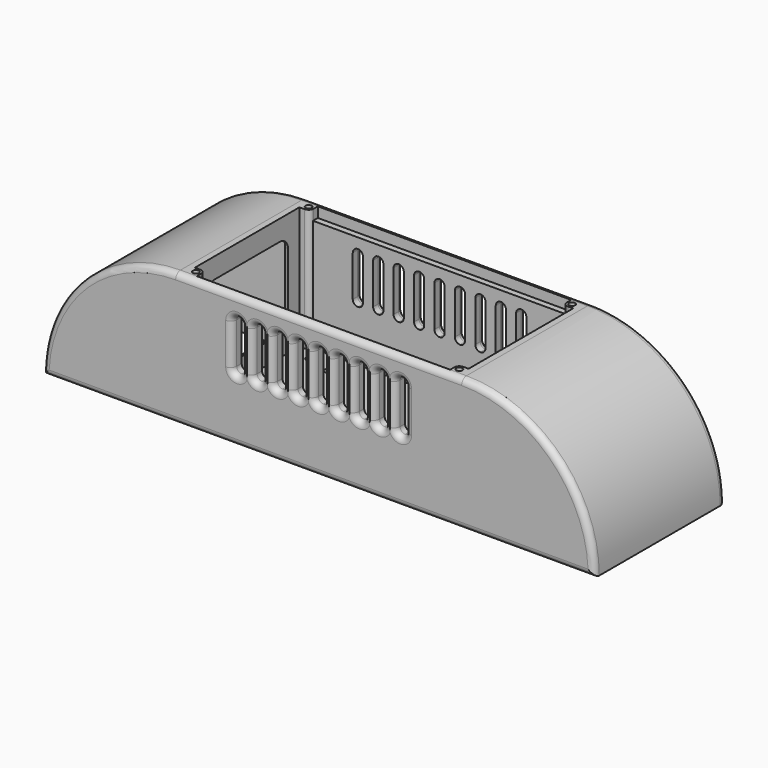
from build123d import *

# Parameters (mm, degrees)
F0_R           = 2.5
F0_R_2         = 1.5
F1_DEPTH       = 5
F0_W           = 140
F0_H           = 80
F2_DEPTH       = 65
F5_DEPTH       = 10
F8_DEPTH       = 10
F9_DEPTH       = 60
F10_DEPTH      = 85
F13_DEPTH      = 80
F14_DEPTH      = 70
F15_T1_DEPTH   = 70
F15_T3_DEPTH   = 285
F15_T5_DEPTH   = 140
F15_T7_DEPTH   = 20
F15_T9_DEPTH   = 70
F15_T11_DEPTH  = 46
F15_T13_DEPTH  = 40
F15_T15_DEPTH  = 30
F15_T17_DEPTH  = 27.5
F15_T20_ANGLE  = 96.6137071956
F15_T22_ANGLE  = 96.6137071956
F15_T24_ANGLE  = 96.6137071956
F15_T26_ANGLE  = 180
F15_T28_ANGLE  = 180
F15_T30_ANGLE  = 180
F15_T32_ANGLE  = 180
F15_T34_ANGLE  = 180
F15_T36_ANGLE  = 180
F15_T38_ANGLE  = 180
F15_T40_ANGLE  = 180
F15_T42_ANGLE  = 180
F15_T44_ANGLE  = 180
F15_T46_ANGLE  = 180
F15_T48_ANGLE  = 180
F15_T50_ANGLE  = 180
F15_T52_ANGLE  = 180
F15_T54_ANGLE  = 180
F15_T56_ANGLE  = 180
F15_T58_ANGLE  = 180
F15_T60_ANGLE  = 180
F15_T62_ANGLE  = 96.6137071956
F15_T64_ANGLE  = 180
F15_T66_ANGLE  = 180
F15_T68_ANGLE  = 180
F15_T70_ANGLE  = 180
F15_T72_ANGLE  = 180
F15_T74_ANGLE  = 180
F15_T76_ANGLE  = 180
F15_T78_ANGLE  = 180
F15_T80_ANGLE  = 180
F15_T82_ANGLE  = 180
F15_T84_ANGLE  = 180
F15_T86_ANGLE  = 180
F15_T88_ANGLE  = 180
F15_T90_ANGLE  = 180
F15_T92_ANGLE  = 180
F15_T94_ANGLE  = 180
F15_T96_ANGLE  = 180
F15_T98_ANGLE  = 180
F15_T100_ANGLE = 90
F15_T102_ANGLE = 90
F15_T104_ANGLE = 90
F15_T106_ANGLE = 90
F15_T108_ANGLE = 90
F15_T110_ANGLE = 90
F15_T112_ANGLE = 90
F15_T114_ANGLE = 90


# Not quite as in the source:
# - a fillet or chamfer that OpenCascade refuses, or shapes differently, is made with other operations: its cross-section is extruded or revolved along the edge and cut away or added


with BuildPart() as f1:
    # F0 (on Top) → F1 (new body)
    with BuildSketch(Plane.XY):
        with BuildLine():
            Line((5.5, 72), (3, 72))
            Line((3, 72), (3, 8))
            Line((3, 8), (5.5, 8))
            ThreePointArc((5.5, 8), (7.0811388301, 7.4364916731), (7.9494897428, 6))
            Line((7.9494897428, 6), (132.0505102572, 6))
            ThreePointArc((132.0505102572, 6), (132.9188611699, 7.4364916731), (134.5, 8))
            Line((134.5, 8), (137, 8))
            Line((137, 8), (137, 72))
            Line((137, 72), (134.5, 72))
            ThreePointArc((134.5, 72), (132.9188611699, 72.5635083269), (132.0505102572, 74))
            Line((132.0505102572, 74), (7.9494897428, 74))
            ThreePointArc((7.9494897428, 74), (7.0811388301, 72.5635083269), (5.5, 72))
        make_face()
        with Locations((13, 13)):
            Circle(F0_R, mode=Mode.SUBTRACT)
        with Locations((31, 15)):
            Circle(F0_R_2, mode=Mode.SUBTRACT)
        with Locations((106, 15)):
            Circle(F0_R_2, mode=Mode.SUBTRACT)
        with Locations((127, 13)):
            Circle(F0_R, mode=Mode.SUBTRACT)
        with Locations((13, 67)):
            Circle(F0_R, mode=Mode.SUBTRACT)
        with Locations((24, 63)):
            Circle(F0_R_2, mode=Mode.SUBTRACT)
        with Locations((106, 63)):
            Circle(F0_R_2, mode=Mode.SUBTRACT)
        with Locations((127, 67)):
            Circle(F0_R, mode=Mode.SUBTRACT)
    extrude(amount=F1_DEPTH)

    # F0 (on Top) → F2 (join)
    with BuildSketch(Plane.XY):
        with Locations((70, 40)):
            Rectangle(F0_W, F0_H)
        with Locations((5.5, 5.5)):
            Circle(F0_R_2, mode=Mode.SUBTRACT)
        with Locations((134.5, 5.5)):
            Circle(F0_R_2, mode=Mode.SUBTRACT)
        with Locations((5.5, 74.5)):
            Circle(F0_R_2, mode=Mode.SUBTRACT)
        with BuildLine():
            Line((3, 8), (3, 72))
            Line((3, 72), (5.5, 72))
            ThreePointArc((5.5, 72), (7.0811388301, 72.5635083269), (7.9494897428, 74))
            ThreePointArc((7.9494897428, 74), (7.9873403825, 74.248727595), (8, 74.5))
            Line((8, 74.5), (8, 77))
            Line((8, 77), (132, 77))
            Line((132, 77), (132, 74.5))
            ThreePointArc((132, 74.5), (132.0126596175, 74.248727595), (132.0505102572, 74))
            ThreePointArc((132.0505102572, 74), (132.9188611699, 72.5635083269), (134.5, 72))
            Line((134.5, 72), (137, 72))
            Line((137, 72), (137, 8))
            Line((137, 8), (134.5, 8))
            ThreePointArc((134.5, 8), (132.9188611699, 7.4364916731), (132.0505102572, 6))
            ThreePointArc((132.0505102572, 6), (132.0126596175, 5.751272405), (132, 5.5))
            Line((132, 5.5), (132, 3))
            Line((132, 3), (8, 3))
            Line((8, 3), (8, 5.5))
            ThreePointArc((8, 5.5), (7.9873403825, 5.751272405), (7.9494897428, 6))
            ThreePointArc((7.9494897428, 6), (7.0811388301, 7.4364916731), (5.5, 8))
            Line((5.5, 8), (3, 8))
        make_face(mode=Mode.SUBTRACT)
        with Locations((134.5, 74.5)):
            Circle(F0_R_2, mode=Mode.SUBTRACT)
    extrude(amount=F2_DEPTH)

    # F4 (on Right) → F5 (cut)
    with BuildSketch(Plane.YZ):
        with BuildLine():
            Line((60, 55), (20, 55))
            ThreePointArc((20, 55), (16.4644660941, 53.5355339059), (15, 50))
            Line((15, 50), (15, 20))
            ThreePointArc((15, 20), (16.4644660941, 16.4644660941), (20, 15))
            Line((20, 15), (60, 15))
            ThreePointArc((60, 15), (63.5355339059, 16.4644660941), (65, 20))
            Line((65, 20), (65, 50))
            ThreePointArc((65, 50), (63.5355339059, 53.5355339059), (60, 55))
        make_face()
    extrude(amount=F5_DEPTH, mode=Mode.SUBTRACT)

    # F7 (on offset) → F8 (cut)
    with BuildSketch(Plane.YZ.offset(140)):
        with BuildLine():
            ThreePointArc((66, 10.5), (67.4142135624, 11.0857864376), (68, 12.5))
            Line((68, 12.5), (68, 40))
            ThreePointArc((68, 40), (67.4142135624, 41.4142135624), (66, 42))
            Line((66, 42), (20, 42))
            ThreePointArc((20, 42), (18.5857864376, 41.4142135624), (18, 40))
            Line((18, 40), (18, 12.5))
            ThreePointArc((18, 12.5), (18.5857864376, 11.0857864376), (20, 10.5))
            Line((20, 10.5), (66, 10.5))
        make_face()
    extrude(amount=-F8_DEPTH, mode=Mode.SUBTRACT)

    # F0 (on Top) → F9 (join)
    with BuildSketch(Plane.XY):
        with BuildLine():
            Line((132.0505102572, 6), (7.9494897428, 6))
            ThreePointArc((7.9494897428, 6), (7.9873403825, 5.751272405), (8, 5.5))
            Line((8, 5.5), (8, 3))
            Line((8, 3), (132, 3))
            Line((132, 3), (132, 5.5))
            ThreePointArc((132, 5.5), (132.0126596175, 5.751272405), (132.0505102572, 6))
        make_face()
        with BuildLine():
            ThreePointArc((8, 74.5), (7.9873403825, 74.248727595), (7.9494897428, 74))
            Line((7.9494897428, 74), (132.0505102572, 74))
            ThreePointArc((132.0505102572, 74), (132.0126596175, 74.248727595), (132, 74.5))
            Line((132, 74.5), (132, 77))
            Line((132, 77), (8, 77))
            Line((8, 77), (8, 74.5))
        make_face()
    extrude(amount=F9_DEPTH)

    # F3 (on Front) → F10 (cut)
    with BuildSketch(Plane.XZ):
        with BuildLine():
            ThreePointArc((30, 30), (31.767766953, 30.732233047), (32.5, 32.5))
            Line((32.5, 32.5), (32.5, 52.5))
            ThreePointArc((32.5, 52.5), (31.767766953, 54.267766953), (30, 55))
            ThreePointArc((30, 55), (28.232233047, 54.267766953), (27.5, 52.5))
            Line((27.5, 52.5), (27.5, 32.5))
            ThreePointArc((27.5, 32.5), (28.232233047, 30.732233047), (30, 30))
        make_face()
        with BuildLine():
            ThreePointArc((40, 30), (41.767766953, 30.732233047), (42.5, 32.5))
            Line((42.5, 32.5), (42.5, 52.5))
            ThreePointArc((42.5, 52.5), (41.767766953, 54.267766953), (40, 55))
            ThreePointArc((40, 55), (38.232233047, 54.267766953), (37.5, 52.5))
            Line((37.5, 52.5), (37.5, 32.5))
            ThreePointArc((37.5, 32.5), (38.232233047, 30.732233047), (40, 30))
        make_face()
        with BuildLine():
            Line((47.5, 52.5), (47.5, 32.5))
            ThreePointArc((47.5, 32.5), (48.232233047, 30.732233047), (50, 30))
            ThreePointArc((50, 30), (51.767766953, 30.732233047), (52.5, 32.5))
            Line((52.5, 32.5), (52.5, 52.5))
            ThreePointArc((52.5, 52.5), (51.767766953, 54.267766953), (50, 55))
            ThreePointArc((50, 55), (48.232233047, 54.267766953), (47.5, 52.5))
        make_face()
        with BuildLine():
            Line((57.5, 52.5), (57.5, 32.5))
            ThreePointArc((57.5, 32.5), (58.232233047, 30.732233047), (60, 30))
            ThreePointArc((60, 30), (61.767766953, 30.732233047), (62.5, 32.5))
            Line((62.5, 32.5), (62.5, 52.5))
            ThreePointArc((62.5, 52.5), (61.767766953, 54.267766953), (60, 55))
            ThreePointArc((60, 55), (58.232233047, 54.267766953), (57.5, 52.5))
        make_face()
        with BuildLine():
            Line((67.5, 52.5), (67.5, 32.5))
            ThreePointArc((67.5, 32.5), (68.232233047, 30.732233047), (70, 30))
            ThreePointArc((70, 30), (71.767766953, 30.732233047), (72.5, 32.5))
            Line((72.5, 32.5), (72.5, 52.5))
            ThreePointArc((72.5, 52.5), (71.767766953, 54.267766953), (70, 55))
            ThreePointArc((70, 55), (68.232233047, 54.267766953), (67.5, 52.5))
        make_face()
        with BuildLine():
            Line((77.5, 52.5), (77.5, 32.5))
            ThreePointArc((77.5, 32.5), (78.232233047, 30.732233047), (80, 30))
            ThreePointArc((80, 30), (81.767766953, 30.732233047), (82.5, 32.5))
            Line((82.5, 32.5), (82.5, 52.5))
            ThreePointArc((82.5, 52.5), (81.767766953, 54.267766953), (80, 55))
            ThreePointArc((80, 55), (78.232233047, 54.267766953), (77.5, 52.5))
        make_face()
        with BuildLine():
            Line((87.5, 52.5), (87.5, 32.5))
            ThreePointArc((87.5, 32.5), (88.232233047, 30.732233047), (90, 30))
            ThreePointArc((90, 30), (91.767766953, 30.732233047), (92.5, 32.5))
            Line((92.5, 32.5), (92.5, 52.5))
            ThreePointArc((92.5, 52.5), (91.767766953, 54.267766953), (90, 55))
            ThreePointArc((90, 55), (88.232233047, 54.267766953), (87.5, 52.5))
        make_face()
        with BuildLine():
            Line((97.5, 52.5), (97.5, 32.5))
            ThreePointArc((97.5, 32.5), (98.232233047, 30.732233047), (100, 30))
            ThreePointArc((100, 30), (101.767766953, 30.732233047), (102.5, 32.5))
            Line((102.5, 32.5), (102.5, 52.5))
            ThreePointArc((102.5, 52.5), (101.767766953, 54.267766953), (100, 55))
            ThreePointArc((100, 55), (98.232233047, 54.267766953), (97.5, 52.5))
        make_face()
        with BuildLine():
            Line((107.5, 52.5), (107.5, 32.5))
            ThreePointArc((107.5, 32.5), (108.232233047, 30.732233047), (110, 30))
            ThreePointArc((110, 30), (111.767766953, 30.732233047), (112.5, 32.5))
            Line((112.5, 32.5), (112.5, 52.5))
            ThreePointArc((112.5, 52.5), (111.767766953, 54.267766953), (110, 55))
            ThreePointArc((110, 55), (108.232233047, 54.267766953), (107.5, 52.5))
        make_face()
    extrude(amount=-F10_DEPTH, mode=Mode.SUBTRACT)

    # F3 (on Front) → F13 (join)
    with BuildSketch(Plane.XZ):
        with BuildLine():
            Line((140, 65), (140, 0))
            Line((140, 0), (205, 0))
            ThreePointArc((205, 0), (185.9619407771, 45.9619407771), (140, 65))
        make_face()
        with BuildLine():
            Line((0, 0), (0, 65))
            ThreePointArc((0, 65), (-45.9619407771, 45.9619407771), (-65, 0))
            Line((-65, 0), (0, 0))
        make_face()
    extrude(amount=-F13_DEPTH)

    # F12 (on offset) → F14 (cut)
    with BuildSketch(Plane.XZ.offset(-5)):
        with BuildLine():
            Line((140, 60), (140, 5))
            Line((140, 5), (145, 5))
            Line((145, 5), (145, 0))
            Line((145, 0), (190, 0))
            Line((190, 0), (190, 5))
            Line((190, 5), (199.7913037155, 5))
            ThreePointArc((199.7913037155, 5), (180.6201920232, 44.1588043316), (140, 60))
        make_face()
        with BuildLine():
            Line((-5, 5), (0, 5))
            Line((0, 5), (0, 60))
            ThreePointArc((0, 60), (-40.6201920232, 44.1588043316), (-59.7913037155, 5))
            Line((-59.7913037155, 5), (-50, 5))
            Line((-50, 5), (-50, 0))
            Line((-50, 0), (-5, 0))
            Line((-5, 0), (-5, 5))
        make_face()
    extrude(amount=-F14_DEPTH, mode=Mode.SUBTRACT)

    # F15: fillet of radius 3 on 102 edges, made by hand

    # F15_s2 → F15_t1 (join)
    with BuildSketch(Plane.XZ.offset(-75)):
        with BuildLine():
            ThreePointArc((199.4061097243, 8.4210526316), (198.701103103, 6.0331697957), (196.4358042381, 5))
            Line((196.4358042381, 5), (199.7913037155, 5))
            ThreePointArc((199.7913037155, 5), (199.6232483429, 6.7132895839), (199.4061097243, 8.4210526316))
        make_face()
        with BuildLine():
            ThreePointArc((-59.4061097243, 8.4210526316), (-58.701103103, 6.0331697957), (-56.4358042381, 5))
            Line((-56.4358042381, 5), (-59.7913037155, 5))
            ThreePointArc((-59.7913037155, 5), (-59.6232483429, 6.7132895839), (-59.4061097243, 8.4210526316))
        make_face()
    extrude(amount=F15_T1_DEPTH)

    # F15_s4 → F15_t3 (cut)
    with BuildSketch(Plane.YZ.offset(-72.5)):
        with BuildLine():
            ThreePointArc((80, 3), (79.1213203436, 0.8786796564), (77, 0))
            Line((77, 0), (80, 0))
            Line((80, 0), (80, 3))
        make_face()
        with BuildLine():
            ThreePointArc((0, 3), (0.8786796564, 0.8786796564), (3, 0))
            Line((3, 0), (0, 0))
            Line((0, 0), (0, 3))
        make_face()
    extrude(amount=F15_T3_DEPTH, mode=Mode.SUBTRACT)

    # F15_s6 → F15_t5 (cut)
    with BuildSketch(Plane.YZ):
        with BuildLine():
            ThreePointArc((77, 65), (79.1213203436, 64.1213203436), (80, 62))
            Line((80, 62), (80, 65))
            Line((80, 65), (77, 65))
        make_face()
        with BuildLine():
            ThreePointArc((3, 65), (0.8786796564, 64.1213203436), (0, 62))
            Line((0, 62), (0, 65))
            Line((0, 65), (3, 65))
        make_face()
    extrude(amount=F15_T5_DEPTH, mode=Mode.SUBTRACT)

    # F15_s8 → F15_t7 (cut)
    with BuildSketch(Plane.XY.offset(32.5)):
        with BuildLine():
            ThreePointArc((104.5, 80), (106.6213203436, 79.1213203436), (107.5, 77))
            Line((107.5, 77), (107.5, 80))
            Line((107.5, 80), (104.5, 80))
        make_face()
        with BuildLine():
            ThreePointArc((115.5, 80), (113.3786796564, 79.1213203436), (112.5, 77))
            Line((112.5, 77), (112.5, 80))
            Line((112.5, 80), (115.5, 80))
        make_face()
        with BuildLine():
            ThreePointArc((94.5, 80), (96.6213203436, 79.1213203436), (97.5, 77))
            Line((97.5, 77), (97.5, 80))
            Line((97.5, 80), (94.5, 80))
        make_face()
        with BuildLine():
            ThreePointArc((105.5, 80), (103.3786796564, 79.1213203436), (102.5, 77))
            Line((102.5, 77), (102.5, 80))
            Line((102.5, 80), (105.5, 80))
        make_face()
        with BuildLine():
            ThreePointArc((84.5, 80), (86.6213203436, 79.1213203436), (87.5, 77))
            Line((87.5, 77), (87.5, 80))
            Line((87.5, 80), (84.5, 80))
        make_face()
        with BuildLine():
            ThreePointArc((95.5, 80), (93.3786796564, 79.1213203436), (92.5, 77))
            Line((92.5, 77), (92.5, 80))
            Line((92.5, 80), (95.5, 80))
        make_face()
        with BuildLine():
            ThreePointArc((74.5, 80), (76.6213203436, 79.1213203436), (77.5, 77))
            Line((77.5, 77), (77.5, 80))
            Line((77.5, 80), (74.5, 80))
        make_face()
        with BuildLine():
            ThreePointArc((85.5, 80), (83.3786796564, 79.1213203436), (82.5, 77))
            Line((82.5, 77), (82.5, 80))
            Line((82.5, 80), (85.5, 80))
        make_face()
        with BuildLine():
            ThreePointArc((64.5, 80), (66.6213203436, 79.1213203436), (67.5, 77))
            Line((67.5, 77), (67.5, 80))
            Line((67.5, 80), (64.5, 80))
        make_face()
        with BuildLine():
            ThreePointArc((75.5, 80), (73.3786796564, 79.1213203436), (72.5, 77))
            Line((72.5, 77), (72.5, 80))
            Line((72.5, 80), (75.5, 80))
        make_face()
        with BuildLine():
            ThreePointArc((54.5, 80), (56.6213203436, 79.1213203436), (57.5, 77))
            Line((57.5, 77), (57.5, 80))
            Line((57.5, 80), (54.5, 80))
        make_face()
        with BuildLine():
            ThreePointArc((65.5, 80), (63.3786796564, 79.1213203436), (62.5, 77))
            Line((62.5, 77), (62.5, 80))
            Line((62.5, 80), (65.5, 80))
        make_face()
        with BuildLine():
            ThreePointArc((44.5, 80), (46.6213203436, 79.1213203436), (47.5, 77))
            Line((47.5, 77), (47.5, 80))
            Line((47.5, 80), (44.5, 80))
        make_face()
        with BuildLine():
            ThreePointArc((55.5, 80), (53.3786796564, 79.1213203436), (52.5, 77))
            Line((52.5, 77), (52.5, 80))
            Line((52.5, 80), (55.5, 80))
        make_face()
        with BuildLine():
            ThreePointArc((45.5, 80), (43.3786796564, 79.1213203436), (42.5, 77))
            Line((42.5, 77), (42.5, 80))
            Line((42.5, 80), (45.5, 80))
        make_face()
        with BuildLine():
            ThreePointArc((34.5, 80), (36.6213203436, 79.1213203436), (37.5, 77))
            Line((37.5, 77), (37.5, 80))
            Line((37.5, 80), (34.5, 80))
        make_face()
        with BuildLine():
            ThreePointArc((35.5, 80), (33.3786796564, 79.1213203436), (32.5, 77))
            Line((32.5, 77), (32.5, 80))
            Line((32.5, 80), (35.5, 80))
        make_face()
        with BuildLine():
            ThreePointArc((24.5, 80), (26.6213203436, 79.1213203436), (27.5, 77))
            Line((27.5, 77), (27.5, 80))
            Line((27.5, 80), (24.5, 80))
        make_face()
        with BuildLine():
            ThreePointArc((107.5, 3), (106.6213203436, 0.8786796564), (104.5, 0))
            Line((104.5, 0), (107.5, 0))
            Line((107.5, 0), (107.5, 3))
        make_face()
        with BuildLine():
            ThreePointArc((112.5, 3), (113.3786796564, 0.8786796564), (115.5, 0))
            Line((115.5, 0), (112.5, 0))
            Line((112.5, 0), (112.5, 3))
        make_face()
        with BuildLine():
            ThreePointArc((32.5, 3), (33.3786796564, 0.8786796564), (35.5, 0))
            Line((35.5, 0), (32.5, 0))
            Line((32.5, 0), (32.5, 3))
        make_face()
        with BuildLine():
            ThreePointArc((27.5, 3), (26.6213203436, 0.8786796564), (24.5, 0))
            Line((24.5, 0), (27.5, 0))
            Line((27.5, 0), (27.5, 3))
        make_face()
        with BuildLine():
            ThreePointArc((42.5, 3), (43.3786796564, 0.8786796564), (45.5, 0))
            Line((45.5, 0), (42.5, 0))
            Line((42.5, 0), (42.5, 3))
        make_face()
        with BuildLine():
            ThreePointArc((37.5, 3), (36.6213203436, 0.8786796564), (34.5, 0))
            Line((34.5, 0), (37.5, 0))
            Line((37.5, 0), (37.5, 3))
        make_face()
        with BuildLine():
            ThreePointArc((47.5, 3), (46.6213203436, 0.8786796564), (44.5, 0))
            Line((44.5, 0), (47.5, 0))
            Line((47.5, 0), (47.5, 3))
        make_face()
        with BuildLine():
            ThreePointArc((52.5, 3), (53.3786796564, 0.8786796564), (55.5, 0))
            Line((55.5, 0), (52.5, 0))
            Line((52.5, 0), (52.5, 3))
        make_face()
        with BuildLine():
            ThreePointArc((57.5, 3), (56.6213203436, 0.8786796564), (54.5, 0))
            Line((54.5, 0), (57.5, 0))
            Line((57.5, 0), (57.5, 3))
        make_face()
        with BuildLine():
            ThreePointArc((62.5, 3), (63.3786796564, 0.8786796564), (65.5, 0))
            Line((65.5, 0), (62.5, 0))
            Line((62.5, 0), (62.5, 3))
        make_face()
        with BuildLine():
            ThreePointArc((67.5, 3), (66.6213203436, 0.8786796564), (64.5, 0))
            Line((64.5, 0), (67.5, 0))
            Line((67.5, 0), (67.5, 3))
        make_face()
        with BuildLine():
            ThreePointArc((72.5, 3), (73.3786796564, 0.8786796564), (75.5, 0))
            Line((75.5, 0), (72.5, 0))
            Line((72.5, 0), (72.5, 3))
        make_face()
        with BuildLine():
            ThreePointArc((77.5, 3), (76.6213203436, 0.8786796564), (74.5, 0))
            Line((74.5, 0), (77.5, 0))
            Line((77.5, 0), (77.5, 3))
        make_face()
        with BuildLine():
            ThreePointArc((82.5, 3), (83.3786796564, 0.8786796564), (85.5, 0))
            Line((85.5, 0), (82.5, 0))
            Line((82.5, 0), (82.5, 3))
        make_face()
        with BuildLine():
            ThreePointArc((87.5, 3), (86.6213203436, 0.8786796564), (84.5, 0))
            Line((84.5, 0), (87.5, 0))
            Line((87.5, 0), (87.5, 3))
        make_face()
        with BuildLine():
            ThreePointArc((92.5, 3), (93.3786796564, 0.8786796564), (95.5, 0))
            Line((95.5, 0), (92.5, 0))
            Line((92.5, 0), (92.5, 3))
        make_face()
        with BuildLine():
            ThreePointArc((97.5, 3), (96.6213203436, 0.8786796564), (94.5, 0))
            Line((94.5, 0), (97.5, 0))
            Line((97.5, 0), (97.5, 3))
        make_face()
        with BuildLine():
            ThreePointArc((102.5, 3), (103.3786796564, 0.8786796564), (105.5, 0))
            Line((105.5, 0), (102.5, 0))
            Line((102.5, 0), (102.5, 3))
        make_face()
    extrude(amount=F15_T7_DEPTH, mode=Mode.SUBTRACT)

    # F15_s10 → F15_t9 (cut)
    with BuildSketch(Plane.XZ.offset(-75)):
        with BuildLine():
            ThreePointArc((190, 2), (190.8786796564, 4.1213203436), (193, 5))
            Line((193, 5), (190, 5))
            Line((190, 5), (190, 2))
        make_face()
        with BuildLine():
            ThreePointArc((-50, 2), (-50.8786796564, 4.1213203436), (-53, 5))
            Line((-53, 5), (-50, 5))
            Line((-50, 5), (-50, 2))
        make_face()
        with BuildLine():
            ThreePointArc((145, 2), (144.1213203436, 4.1213203436), (142, 5))
            Line((142, 5), (145, 5))
            Line((145, 5), (145, 2))
        make_face()
        with BuildLine():
            ThreePointArc((-5, 2), (-4.1213203436, 4.1213203436), (-2, 5))
            Line((-2, 5), (-5, 5))
            Line((-5, 5), (-5, 2))
        make_face()
    extrude(amount=F15_T9_DEPTH, mode=Mode.SUBTRACT)

    # F15_s12 → F15_t11 (cut)
    with BuildSketch(Plane.XZ.offset(-66)):
        with BuildLine():
            ThreePointArc((137, 10.5), (139.1213203436, 9.6213203436), (140, 7.5))
            Line((140, 7.5), (140, 10.5))
            Line((140, 10.5), (137, 10.5))
        make_face()
        with BuildLine():
            ThreePointArc((137, 42), (139.1213203436, 42.8786796564), (140, 45))
            Line((140, 45), (140, 42))
            Line((140, 42), (137, 42))
        make_face()
    extrude(amount=F15_T11_DEPTH, mode=Mode.SUBTRACT)

    # F15_s14 → F15_t13 (cut)
    with BuildSketch(Plane.XZ.offset(-60)):
        with BuildLine():
            ThreePointArc((3, 15), (0.8786796564, 14.1213203436), (0, 12))
            Line((0, 12), (0, 15))
            Line((0, 15), (3, 15))
        make_face()
        with BuildLine():
            ThreePointArc((3, 55), (0.8786796564, 55.8786796564), (0, 58))
            Line((0, 58), (0, 55))
            Line((0, 55), (3, 55))
        make_face()
    extrude(amount=F15_T13_DEPTH, mode=Mode.SUBTRACT)

    # F15_s16 → F15_t15 (cut)
    with BuildSketch(Plane.XY.offset(20)):
        with BuildLine():
            ThreePointArc((3, 65), (0.8786796564, 65.8786796564), (0, 68))
            Line((0, 68), (0, 65))
            Line((0, 65), (3, 65))
        make_face()
        with BuildLine():
            ThreePointArc((3, 15), (0.8786796564, 14.1213203436), (0, 12))
            Line((0, 12), (0, 15))
            Line((0, 15), (3, 15))
        make_face()
    extrude(amount=F15_T15_DEPTH, mode=Mode.SUBTRACT)

    # F15_s18 → F15_t17 (cut)
    with BuildSketch(Plane.XY.offset(12.5)):
        with BuildLine():
            ThreePointArc((137, 68), (139.1213203436, 68.8786796564), (140, 71))
            Line((140, 71), (140, 68))
            Line((140, 68), (137, 68))
        make_face()
        with BuildLine():
            ThreePointArc((137, 18), (139.1213203436, 17.1213203436), (140, 15))
            Line((140, 15), (140, 18))
            Line((140, 18), (137, 18))
        make_face()
    extrude(amount=F15_T17_DEPTH, mode=Mode.SUBTRACT)

    # F15_s19 → F15_t20 (revolve, cut)
    with BuildSketch(Plane.YZ):
        with BuildLine():
            ThreePointArc((3, 65), (0.8786796564, 64.1213203436), (0, 62))
            Line((0, 62), (0, 65))
            Line((0, 65), (3, 65))
        make_face()
    revolve(axis=Axis((0, 0, 0), (0, -1, 0)), revolution_arc=F15_T20_ANGLE, mode=Mode.SUBTRACT)

    # F15_s21 → F15_t22 (revolve, cut)
    with BuildSketch(Plane.YZ):
        with BuildLine():
            ThreePointArc((77, 65), (79.1213203436, 64.1213203436), (80, 62))
            Line((80, 62), (80, 65))
            Line((80, 65), (77, 65))
        make_face()
    revolve(axis=Axis((0, 80, 0), (0, -1, 0)), revolution_arc=F15_T22_ANGLE, mode=Mode.SUBTRACT)

    # F15_s23 → F15_t24 (revolve, cut)
    with BuildSketch(Plane(origin=(1.8571327546, 0, 16.0171671522), x_dir=(0, 1, 0), z_dir=(-0.1151747974, 0, -0.9933452401))):
        with BuildLine():
            ThreePointArc((77, 204.0683336146), (79.1213203436, 203.1896539582), (80, 201.0683336146))
            Line((80, 201.0683336146), (80, 204.0683336146))
            Line((80, 204.0683336146), (77, 204.0683336146))
        make_face()
    revolve(axis=Axis((140, 80, 0), (0, -1, 0)), revolution_arc=F15_T24_ANGLE, mode=Mode.SUBTRACT)

    # F15_s25 → F15_t26 (revolve, cut)
    with BuildSketch(Plane.XY.offset(52.5)):
        with BuildLine():
            ThreePointArc((115.5, 80), (113.3786796564, 79.1213203436), (112.5, 77))
            Line((112.5, 77), (112.5, 80))
            Line((112.5, 80), (115.5, 80))
        make_face()
    revolve(axis=Axis((110, 80, 52.5), (0, -1, 0)), revolution_arc=F15_T26_ANGLE, mode=Mode.SUBTRACT)

    # F15_s27 → F15_t28 (revolve, cut)
    with BuildSketch(Plane.XY.offset(32.5)):
        with BuildLine():
            ThreePointArc((104.5, 80), (106.6213203436, 79.1213203436), (107.5, 77))
            Line((107.5, 77), (107.5, 80))
            Line((107.5, 80), (104.5, 80))
        make_face()
    revolve(axis=Axis((110, 80, 32.5), (0, -1, 0)), revolution_arc=F15_T28_ANGLE, mode=Mode.SUBTRACT)

    # F15_s29 → F15_t30 (revolve, cut)
    with BuildSketch(Plane.XY.offset(52.5)):
        with BuildLine():
            ThreePointArc((105.5, 80), (103.3786796564, 79.1213203436), (102.5, 77))
            Line((102.5, 77), (102.5, 80))
            Line((102.5, 80), (105.5, 80))
        make_face()
    revolve(axis=Axis((100, 80, 52.5), (0, -1, 0)), revolution_arc=F15_T30_ANGLE, mode=Mode.SUBTRACT)

    # F15_s31 → F15_t32 (revolve, cut)
    with BuildSketch(Plane.XY.offset(32.5)):
        with BuildLine():
            ThreePointArc((94.5, 80), (96.6213203436, 79.1213203436), (97.5, 77))
            Line((97.5, 77), (97.5, 80))
            Line((97.5, 80), (94.5, 80))
        make_face()
    revolve(axis=Axis((100, 80, 32.5), (0, -1, 0)), revolution_arc=F15_T32_ANGLE, mode=Mode.SUBTRACT)

    # F15_s33 → F15_t34 (revolve, cut)
    with BuildSketch(Plane.XY.offset(52.5)):
        with BuildLine():
            ThreePointArc((95.5, 80), (93.3786796564, 79.1213203436), (92.5, 77))
            Line((92.5, 77), (92.5, 80))
            Line((92.5, 80), (95.5, 80))
        make_face()
    revolve(axis=Axis((90, 80, 52.5), (0, -1, 0)), revolution_arc=F15_T34_ANGLE, mode=Mode.SUBTRACT)

    # F15_s35 → F15_t36 (revolve, cut)
    with BuildSketch(Plane.XY.offset(32.5)):
        with BuildLine():
            ThreePointArc((84.5, 80), (86.6213203436, 79.1213203436), (87.5, 77))
            Line((87.5, 77), (87.5, 80))
            Line((87.5, 80), (84.5, 80))
        make_face()
    revolve(axis=Axis((90, 80, 32.5), (0, -1, 0)), revolution_arc=F15_T36_ANGLE, mode=Mode.SUBTRACT)

    # F15_s37 → F15_t38 (revolve, cut)
    with BuildSketch(Plane.XY.offset(52.5)):
        with BuildLine():
            ThreePointArc((85.5, 80), (83.3786796564, 79.1213203436), (82.5, 77))
            Line((82.5, 77), (82.5, 80))
            Line((82.5, 80), (85.5, 80))
        make_face()
    revolve(axis=Axis((80, 80, 52.5), (0, -1, 0)), revolution_arc=F15_T38_ANGLE, mode=Mode.SUBTRACT)

    # F15_s39 → F15_t40 (revolve, cut)
    with BuildSketch(Plane.XY.offset(32.5)):
        with BuildLine():
            ThreePointArc((74.5, 80), (76.6213203436, 79.1213203436), (77.5, 77))
            Line((77.5, 77), (77.5, 80))
            Line((77.5, 80), (74.5, 80))
        make_face()
    revolve(axis=Axis((80, 80, 32.5), (0, -1, 0)), revolution_arc=F15_T40_ANGLE, mode=Mode.SUBTRACT)

    # F15_s41 → F15_t42 (revolve, cut)
    with BuildSketch(Plane.XY.offset(52.5)):
        with BuildLine():
            ThreePointArc((75.5, 80), (73.3786796564, 79.1213203436), (72.5, 77))
            Line((72.5, 77), (72.5, 80))
            Line((72.5, 80), (75.5, 80))
        make_face()
    revolve(axis=Axis((70, 80, 52.5), (0, -1, 0)), revolution_arc=F15_T42_ANGLE, mode=Mode.SUBTRACT)

    # F15_s43 → F15_t44 (revolve, cut)
    with BuildSketch(Plane.XY.offset(32.5)):
        with BuildLine():
            ThreePointArc((64.5, 80), (66.6213203436, 79.1213203436), (67.5, 77))
            Line((67.5, 77), (67.5, 80))
            Line((67.5, 80), (64.5, 80))
        make_face()
    revolve(axis=Axis((70, 80, 32.5), (0, -1, 0)), revolution_arc=F15_T44_ANGLE, mode=Mode.SUBTRACT)

    # F15_s45 → F15_t46 (revolve, cut)
    with BuildSketch(Plane.XY.offset(52.5)):
        with BuildLine():
            ThreePointArc((65.5, 80), (63.3786796564, 79.1213203436), (62.5, 77))
            Line((62.5, 77), (62.5, 80))
            Line((62.5, 80), (65.5, 80))
        make_face()
    revolve(axis=Axis((60, 80, 52.5), (0, -1, 0)), revolution_arc=F15_T46_ANGLE, mode=Mode.SUBTRACT)

    # F15_s47 → F15_t48 (revolve, cut)
    with BuildSketch(Plane.XY.offset(32.5)):
        with BuildLine():
            ThreePointArc((54.5, 80), (56.6213203436, 79.1213203436), (57.5, 77))
            Line((57.5, 77), (57.5, 80))
            Line((57.5, 80), (54.5, 80))
        make_face()
    revolve(axis=Axis((60, 80, 32.5), (0, -1, 0)), revolution_arc=F15_T48_ANGLE, mode=Mode.SUBTRACT)

    # F15_s49 → F15_t50 (revolve, cut)
    with BuildSketch(Plane.XY.offset(52.5)):
        with BuildLine():
            ThreePointArc((55.5, 80), (53.3786796564, 79.1213203436), (52.5, 77))
            Line((52.5, 77), (52.5, 80))
            Line((52.5, 80), (55.5, 80))
        make_face()
    revolve(axis=Axis((50, 80, 52.5), (0, -1, 0)), revolution_arc=F15_T50_ANGLE, mode=Mode.SUBTRACT)

    # F15_s51 → F15_t52 (revolve, cut)
    with BuildSketch(Plane.XY.offset(32.5)):
        with BuildLine():
            ThreePointArc((44.5, 80), (46.6213203436, 79.1213203436), (47.5, 77))
            Line((47.5, 77), (47.5, 80))
            Line((47.5, 80), (44.5, 80))
        make_face()
    revolve(axis=Axis((50, 80, 32.5), (0, -1, 0)), revolution_arc=F15_T52_ANGLE, mode=Mode.SUBTRACT)

    # F15_s53 → F15_t54 (revolve, cut)
    with BuildSketch(Plane.XY.offset(32.5)):
        with BuildLine():
            ThreePointArc((34.5, 80), (36.6213203436, 79.1213203436), (37.5, 77))
            Line((37.5, 77), (37.5, 80))
            Line((37.5, 80), (34.5, 80))
        make_face()
    revolve(axis=Axis((40, 80, 32.5), (0, -1, 0)), revolution_arc=F15_T54_ANGLE, mode=Mode.SUBTRACT)

    # F15_s55 → F15_t56 (revolve, cut)
    with BuildSketch(Plane.XY.offset(52.5)):
        with BuildLine():
            ThreePointArc((45.5, 80), (43.3786796564, 79.1213203436), (42.5, 77))
            Line((42.5, 77), (42.5, 80))
            Line((42.5, 80), (45.5, 80))
        make_face()
    revolve(axis=Axis((40, 80, 52.5), (0, -1, 0)), revolution_arc=F15_T56_ANGLE, mode=Mode.SUBTRACT)

    # F15_s57 → F15_t58 (revolve, cut)
    with BuildSketch(Plane.XY.offset(32.5)):
        with BuildLine():
            ThreePointArc((24.5, 80), (26.6213203436, 79.1213203436), (27.5, 77))
            Line((27.5, 77), (27.5, 80))
            Line((27.5, 80), (24.5, 80))
        make_face()
    revolve(axis=Axis((30, 80, 32.5), (0, -1, 0)), revolution_arc=F15_T58_ANGLE, mode=Mode.SUBTRACT)

    # F15_s59 → F15_t60 (revolve, cut)
    with BuildSketch(Plane.XY.offset(52.5)):
        with BuildLine():
            ThreePointArc((35.5, 80), (33.3786796564, 79.1213203436), (32.5, 77))
            Line((32.5, 77), (32.5, 80))
            Line((32.5, 80), (35.5, 80))
        make_face()
    revolve(axis=Axis((30, 80, 52.5), (0, -1, 0)), revolution_arc=F15_T60_ANGLE, mode=Mode.SUBTRACT)

    # F15_s61 → F15_t62 (revolve, cut)
    with BuildSketch(Plane(origin=(1.8571327546, 0, 16.0171671522), x_dir=(0, 1, 0), z_dir=(-0.1151747974, 0, -0.9933452401))):
        with BuildLine():
            ThreePointArc((0, 201.0683336146), (0.8786796564, 203.1896539582), (3, 204.0683336146))
            Line((3, 204.0683336146), (0, 204.0683336146))
            Line((0, 204.0683336146), (0, 201.0683336146))
        make_face()
    revolve(axis=Axis((140, 0, 0), (0, -1, 0)), revolution_arc=F15_T62_ANGLE, mode=Mode.SUBTRACT)

    # F15_s63 → F15_t64 (revolve, cut)
    with BuildSketch(Plane.XY.offset(52.5)):
        with BuildLine():
            ThreePointArc((112.5, 3), (113.3786796564, 0.8786796564), (115.5, 0))
            Line((115.5, 0), (112.5, 0))
            Line((112.5, 0), (112.5, 3))
        make_face()
    revolve(axis=Axis((110, 0, 52.5), (0, -1, 0)), revolution_arc=F15_T64_ANGLE, mode=Mode.SUBTRACT)

    # F15_s65 → F15_t66 (revolve, cut)
    with BuildSketch(Plane.XY.offset(32.5)):
        with BuildLine():
            ThreePointArc((107.5, 3), (106.6213203436, 0.8786796564), (104.5, 0))
            Line((104.5, 0), (107.5, 0))
            Line((107.5, 0), (107.5, 3))
        make_face()
    revolve(axis=Axis((110, 0, 32.5), (0, -1, 0)), revolution_arc=F15_T66_ANGLE, mode=Mode.SUBTRACT)

    # F15_s67 → F15_t68 (revolve, cut)
    with BuildSketch(Plane.XY.offset(32.5)):
        with BuildLine():
            ThreePointArc((27.5, 3), (26.6213203436, 0.8786796564), (24.5, 0))
            Line((24.5, 0), (27.5, 0))
            Line((27.5, 0), (27.5, 3))
        make_face()
    revolve(axis=Axis((30, 0, 32.5), (0, -1, 0)), revolution_arc=F15_T68_ANGLE, mode=Mode.SUBTRACT)

    # F15_s69 → F15_t70 (revolve, cut)
    with BuildSketch(Plane.XY.offset(52.5)):
        with BuildLine():
            ThreePointArc((32.5, 3), (33.3786796564, 0.8786796564), (35.5, 0))
            Line((35.5, 0), (32.5, 0))
            Line((32.5, 0), (32.5, 3))
        make_face()
    revolve(axis=Axis((30, 0, 52.5), (0, -1, 0)), revolution_arc=F15_T70_ANGLE, mode=Mode.SUBTRACT)

    # F15_s71 → F15_t72 (revolve, cut)
    with BuildSketch(Plane.XY.offset(32.5)):
        with BuildLine():
            ThreePointArc((37.5, 3), (36.6213203436, 0.8786796564), (34.5, 0))
            Line((34.5, 0), (37.5, 0))
            Line((37.5, 0), (37.5, 3))
        make_face()
    revolve(axis=Axis((40, 0, 32.5), (0, -1, 0)), revolution_arc=F15_T72_ANGLE, mode=Mode.SUBTRACT)

    # F15_s73 → F15_t74 (revolve, cut)
    with BuildSketch(Plane.XY.offset(52.5)):
        with BuildLine():
            ThreePointArc((42.5, 3), (43.3786796564, 0.8786796564), (45.5, 0))
            Line((45.5, 0), (42.5, 0))
            Line((42.5, 0), (42.5, 3))
        make_face()
    revolve(axis=Axis((40, 0, 52.5), (0, -1, 0)), revolution_arc=F15_T74_ANGLE, mode=Mode.SUBTRACT)

    # F15_s75 → F15_t76 (revolve, cut)
    with BuildSketch(Plane.XY.offset(52.5)):
        with BuildLine():
            ThreePointArc((52.5, 3), (53.3786796564, 0.8786796564), (55.5, 0))
            Line((55.5, 0), (52.5, 0))
            Line((52.5, 0), (52.5, 3))
        make_face()
    revolve(axis=Axis((50, 0, 52.5), (0, -1, 0)), revolution_arc=F15_T76_ANGLE, mode=Mode.SUBTRACT)

    # F15_s77 → F15_t78 (revolve, cut)
    with BuildSketch(Plane.XY.offset(32.5)):
        with BuildLine():
            ThreePointArc((47.5, 3), (46.6213203436, 0.8786796564), (44.5, 0))
            Line((44.5, 0), (47.5, 0))
            Line((47.5, 0), (47.5, 3))
        make_face()
    revolve(axis=Axis((50, 0, 32.5), (0, -1, 0)), revolution_arc=F15_T78_ANGLE, mode=Mode.SUBTRACT)

    # F15_s79 → F15_t80 (revolve, cut)
    with BuildSketch(Plane.XY.offset(52.5)):
        with BuildLine():
            ThreePointArc((62.5, 3), (63.3786796564, 0.8786796564), (65.5, 0))
            Line((65.5, 0), (62.5, 0))
            Line((62.5, 0), (62.5, 3))
        make_face()
    revolve(axis=Axis((60, 0, 52.5), (0, -1, 0)), revolution_arc=F15_T80_ANGLE, mode=Mode.SUBTRACT)

    # F15_s81 → F15_t82 (revolve, cut)
    with BuildSketch(Plane.XY.offset(32.5)):
        with BuildLine():
            ThreePointArc((57.5, 3), (56.6213203436, 0.8786796564), (54.5, 0))
            Line((54.5, 0), (57.5, 0))
            Line((57.5, 0), (57.5, 3))
        make_face()
    revolve(axis=Axis((60, 0, 32.5), (0, -1, 0)), revolution_arc=F15_T82_ANGLE, mode=Mode.SUBTRACT)

    # F15_s83 → F15_t84 (revolve, cut)
    with BuildSketch(Plane.XY.offset(52.5)):
        with BuildLine():
            ThreePointArc((72.5, 3), (73.3786796564, 0.8786796564), (75.5, 0))
            Line((75.5, 0), (72.5, 0))
            Line((72.5, 0), (72.5, 3))
        make_face()
    revolve(axis=Axis((70, 0, 52.5), (0, -1, 0)), revolution_arc=F15_T84_ANGLE, mode=Mode.SUBTRACT)

    # F15_s85 → F15_t86 (revolve, cut)
    with BuildSketch(Plane.XY.offset(32.5)):
        with BuildLine():
            ThreePointArc((67.5, 3), (66.6213203436, 0.8786796564), (64.5, 0))
            Line((64.5, 0), (67.5, 0))
            Line((67.5, 0), (67.5, 3))
        make_face()
    revolve(axis=Axis((70, 0, 32.5), (0, -1, 0)), revolution_arc=F15_T86_ANGLE, mode=Mode.SUBTRACT)

    # F15_s87 → F15_t88 (revolve, cut)
    with BuildSketch(Plane.XY.offset(52.5)):
        with BuildLine():
            ThreePointArc((82.5, 3), (83.3786796564, 0.8786796564), (85.5, 0))
            Line((85.5, 0), (82.5, 0))
            Line((82.5, 0), (82.5, 3))
        make_face()
    revolve(axis=Axis((80, 0, 52.5), (0, -1, 0)), revolution_arc=F15_T88_ANGLE, mode=Mode.SUBTRACT)

    # F15_s89 → F15_t90 (revolve, cut)
    with BuildSketch(Plane.XY.offset(32.5)):
        with BuildLine():
            ThreePointArc((77.5, 3), (76.6213203436, 0.8786796564), (74.5, 0))
            Line((74.5, 0), (77.5, 0))
            Line((77.5, 0), (77.5, 3))
        make_face()
    revolve(axis=Axis((80, 0, 32.5), (0, -1, 0)), revolution_arc=F15_T90_ANGLE, mode=Mode.SUBTRACT)

    # F15_s91 → F15_t92 (revolve, cut)
    with BuildSketch(Plane.XY.offset(52.5)):
        with BuildLine():
            ThreePointArc((92.5, 3), (93.3786796564, 0.8786796564), (95.5, 0))
            Line((95.5, 0), (92.5, 0))
            Line((92.5, 0), (92.5, 3))
        make_face()
    revolve(axis=Axis((90, 0, 52.5), (0, -1, 0)), revolution_arc=F15_T92_ANGLE, mode=Mode.SUBTRACT)

    # F15_s93 → F15_t94 (revolve, cut)
    with BuildSketch(Plane.XY.offset(32.5)):
        with BuildLine():
            ThreePointArc((87.5, 3), (86.6213203436, 0.8786796564), (84.5, 0))
            Line((84.5, 0), (87.5, 0))
            Line((87.5, 0), (87.5, 3))
        make_face()
    revolve(axis=Axis((90, 0, 32.5), (0, -1, 0)), revolution_arc=F15_T94_ANGLE, mode=Mode.SUBTRACT)

    # F15_s95 → F15_t96 (revolve, cut)
    with BuildSketch(Plane.XY.offset(52.5)):
        with BuildLine():
            ThreePointArc((102.5, 3), (103.3786796564, 0.8786796564), (105.5, 0))
            Line((105.5, 0), (102.5, 0))
            Line((102.5, 0), (102.5, 3))
        make_face()
    revolve(axis=Axis((100, 0, 52.5), (0, -1, 0)), revolution_arc=F15_T96_ANGLE, mode=Mode.SUBTRACT)

    # F15_s97 → F15_t98 (revolve, cut)
    with BuildSketch(Plane.XY.offset(32.5)):
        with BuildLine():
            ThreePointArc((97.5, 3), (96.6213203436, 0.8786796564), (94.5, 0))
            Line((94.5, 0), (97.5, 0))
            Line((97.5, 0), (97.5, 3))
        make_face()
    revolve(axis=Axis((100, 0, 32.5), (0, -1, 0)), revolution_arc=F15_T98_ANGLE, mode=Mode.SUBTRACT)

    # F15_s99 → F15_t100 (revolve, cut)
    with BuildSketch(Plane.XY.offset(50)):
        with BuildLine():
            ThreePointArc((3, 65), (0.8786796564, 65.8786796564), (0, 68))
            Line((0, 68), (0, 65))
            Line((0, 65), (3, 65))
        make_face()
    revolve(axis=Axis((0, 60, 50), (1, 0, 0)), revolution_arc=F15_T100_ANGLE, mode=Mode.SUBTRACT)

    # F15_s101 → F15_t102 (revolve, cut)
    with BuildSketch(Plane.XZ.offset(-60)):
        with BuildLine():
            ThreePointArc((3, 15), (0.8786796564, 14.1213203436), (0, 12))
            Line((0, 12), (0, 15))
            Line((0, 15), (3, 15))
        make_face()
    revolve(axis=Axis((0, 60, 20), (1, 0, 0)), revolution_arc=F15_T102_ANGLE, mode=Mode.SUBTRACT)

    # F15_s103 → F15_t104 (revolve, cut)
    with BuildSketch(Plane.XY.offset(20)):
        with BuildLine():
            ThreePointArc((3, 15), (0.8786796564, 14.1213203436), (0, 12))
            Line((0, 12), (0, 15))
            Line((0, 15), (3, 15))
        make_face()
    revolve(axis=Axis((0, 20, 20), (1, 0, 0)), revolution_arc=F15_T104_ANGLE, mode=Mode.SUBTRACT)

    # F15_s105 → F15_t106 (revolve, cut)
    with BuildSketch(Plane.XZ.offset(-20)):
        with BuildLine():
            ThreePointArc((3, 55), (0.8786796564, 55.8786796564), (0, 58))
            Line((0, 58), (0, 55))
            Line((0, 55), (3, 55))
        make_face()
    revolve(axis=Axis((0, 20, 50), (1, 0, 0)), revolution_arc=F15_T106_ANGLE, mode=Mode.SUBTRACT)

    # F15_s107 → F15_t108 (revolve, cut)
    with BuildSketch(Plane.XZ.offset(-66)):
        with BuildLine():
            ThreePointArc((137, 10.5), (139.1213203436, 9.6213203436), (140, 7.5))
            Line((140, 7.5), (140, 10.5))
            Line((140, 10.5), (137, 10.5))
        make_face()
    revolve(axis=Axis((140, 66, 12.5), (1, 0, 0)), revolution_arc=F15_T108_ANGLE, mode=Mode.SUBTRACT)

    # F15_s109 → F15_t110 (revolve, cut)
    with BuildSketch(Plane.XY.offset(40)):
        with BuildLine():
            ThreePointArc((137, 68), (139.1213203436, 68.8786796564), (140, 71))
            Line((140, 71), (140, 68))
            Line((140, 68), (137, 68))
        make_face()
    revolve(axis=Axis((140, 66, 40), (1, 0, 0)), revolution_arc=F15_T110_ANGLE, mode=Mode.SUBTRACT)

    # F15_s111 → F15_t112 (revolve, cut)
    with BuildSketch(Plane.XZ.offset(-20)):
        with BuildLine():
            ThreePointArc((137, 42), (139.1213203436, 42.8786796564), (140, 45))
            Line((140, 45), (140, 42))
            Line((140, 42), (137, 42))
        make_face()
    revolve(axis=Axis((140, 20, 40), (1, 0, 0)), revolution_arc=F15_T112_ANGLE, mode=Mode.SUBTRACT)

    # F15_s113 → F15_t114 (revolve, cut)
    with BuildSketch(Plane.XY.offset(12.5)):
        with BuildLine():
            ThreePointArc((137, 18), (139.1213203436, 17.1213203436), (140, 15))
            Line((140, 15), (140, 18))
            Line((140, 18), (137, 18))
        make_face()
    revolve(axis=Axis((140, 20, 12.5), (1, 0, 0)), revolution_arc=F15_T114_ANGLE, mode=Mode.SUBTRACT)


solid = f1.part
